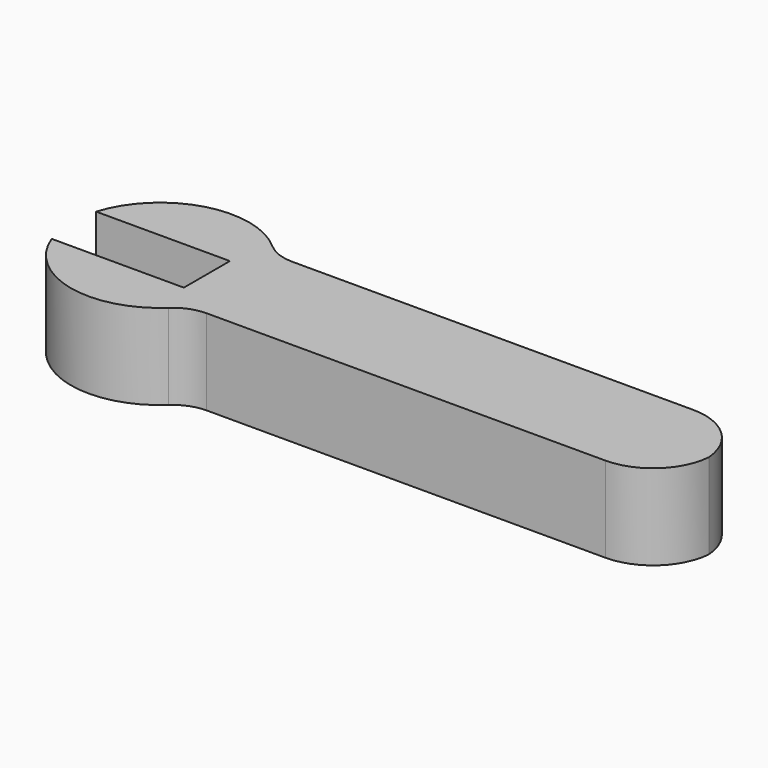
from build123d import *

# Parameters (mm, degrees)
F1_DEPTH    = 25.4
F3_DEPTH    = 38.1
F4_R        = 12.7
F5_R        = 12.7
F6_T1_DEPTH = 114.3


# Not quite as in the source:
# - a fillet or chamfer that OpenCascade refuses, or shapes differently, is made with other operations: its cross-section is extruded or revolved along the edge and cut away or added


with BuildPart() as f1:
    # F0 (on Top) → F1 (new body)
    with BuildSketch(Plane.XY):
        with BuildLine():
            Line((-77.2201499837, 16.618498601), (-92.2268889844, 16.618498601))
            Line((-92.2268889844, 16.618498601), (-92.2268889844, -15.9945080916))
            Line((-92.2268889844, -15.9945080916), (-76.7317300981, -15.9945080916))
            ThreePointArc((-76.7317300981, -15.9945080916), (-72.7314875025, -8.4378237077), (-71.3499844152, 0))
            ThreePointArc((-71.3499844152, 0), (-72.8606518933, 8.8123966597), (-77.2201499837, 16.618498601))
        make_face()
        with BuildLine():
            Line((64.9677813053, 16.618498601), (-77.2201499837, 16.618498601))
            ThreePointArc((-77.2201499837, 16.618498601), (-72.8606518933, 8.8123966597), (-71.3499844152, 0))
            ThreePointArc((-71.3499844152, 0), (-72.7314875025, -8.4378237077), (-76.7317300981, -15.9945080916))
            Line((-76.7317300981, -15.9945080916), (64.9677813053, -15.9945080916))
            Line((64.9677813053, -15.9945080916), (64.9677813053, 16.618498601))
        make_face()
        with BuildLine():
            Line((-92.2268889844, -15.9945080916), (-92.2268889844, 16.618498601))
            Line((-92.2268889844, 16.618498601), (-77.2201499837, 16.618498601))
            ThreePointArc((-77.2201499837, 16.618498601), (-124.2643223617, -0.3962064299), (-76.7317300981, -15.9945080916))
            Line((-76.7317300981, -15.9945080916), (-92.2268889844, -15.9945080916))
        make_face()
    extrude(amount=F1_DEPTH)

    # F2 (on face) → F3 (cut)
    with BuildSketch(Plane.XY.offset(25.4)):
        with BuildLine():
            Line((-83.348184824, 7.8462203965), (-123.0771370274, 7.8462203965))
            ThreePointArc((-123.0771370274, 7.8462203965), (-124.2569046236, -0.741220082), (-122.5980357113, -9.2491069809))
            Line((-122.5980357113, -9.2491069809), (-83.348184824, -9.2491069809))
            Line((-83.348184824, -9.2491069809), (-83.348184824, 7.8462203965))
        make_face()
        with BuildLine():
            Line((-123.0771370274, 7.8462203965), (-131.8430900574, 7.8462203965))
            Line((-131.8430900574, 7.8462203965), (-131.8430900574, -9.2491069809))
            Line((-131.8430900574, -9.2491069809), (-122.5980357113, -9.2491069809))
            ThreePointArc((-122.5980357113, -9.2491069809), (-124.2569046236, -0.741220082), (-123.0771370274, 7.8462203965))
        make_face()
    extrude(amount=-F3_DEPTH, mode=Mode.SUBTRACT)

    # F4
    f4_edges = [f1.edges().sort_by_distance(p)[0] for p in [
        (-77.22015, 16.618499, 12.7),
    ]]
    fillet(f4_edges, radius=F4_R)

    # F5
    f5_edges = [f1.edges().sort_by_distance(p)[0] for p in [
        (-76.73173, -15.994508, 12.7),
    ]]
    fillet(f5_edges, radius=F5_R)

    # F6: fillet of radius 17.78 on 2 edges, made by hand

    # F6_s2 → F6_t1 (cut)
    with BuildSketch(Plane.XY.offset(-44.45)):
        with BuildLine():
            ThreePointArc((64.9677813053, -1.161501399), (59.7601398748, 11.4108571705), (47.1877813053, 16.618498601))
            Line((47.1877813053, 16.618498601), (64.9677813053, 16.618498601))
            Line((64.9677813053, 16.618498601), (64.9677813053, -1.161501399))
        make_face()
        with BuildLine():
            ThreePointArc((47.1877813053, -15.9945080916), (59.7601398748, -10.7868666611), (64.9677813053, 1.7854919084))
            Line((64.9677813053, 1.7854919084), (64.9677813053, -15.9945080916))
            Line((64.9677813053, -15.9945080916), (47.1877813053, -15.9945080916))
        make_face()
    extrude(amount=F6_T1_DEPTH, mode=Mode.SUBTRACT)


solid = f1.part
